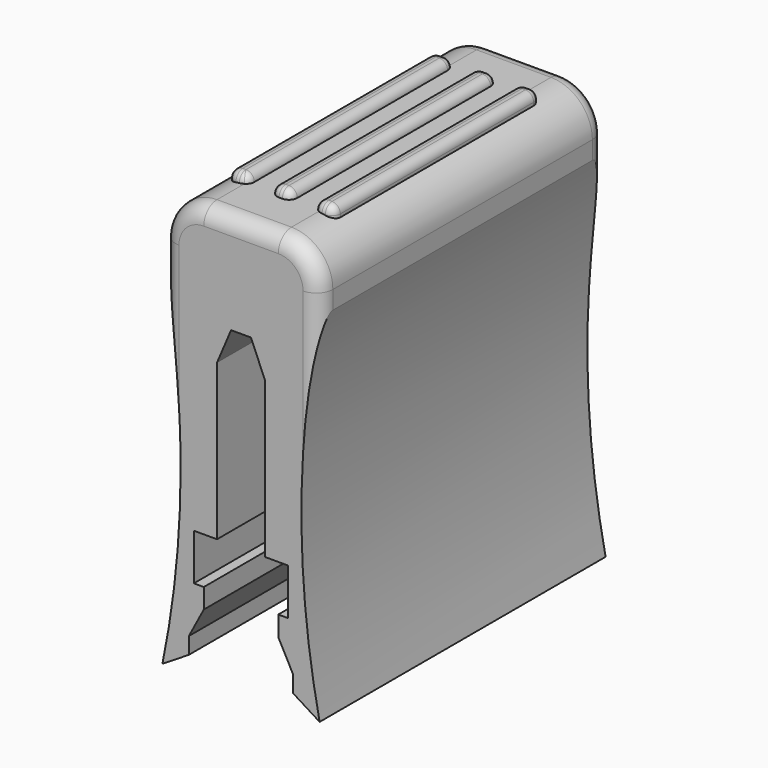
from build123d import *

# Parameters (mm, degrees)
F1_DEPTH = 21.6
F2_R     = 1
F4_DEPTH = 0.5
F5_R     = 0.49999


# Not quite as in the source:
# - a fillet or chamfer is up to 0.001 mm smaller than in the source, because OpenCascade refuses the exact size


with BuildPart() as f1:
    # F0 (on Front) → F1 (new body)
    with BuildSketch(Plane.XZ):
        with BuildLine():
            ThreePointArc((4.75, 10.05), (4.017766953, 11.817766953), (2.25, 12.55))
            Line((2.25, 12.55), (-2.25, 12.55))
            ThreePointArc((-2.25, 12.55), (-4.017766953, 11.817766953), (-4.75, 10.05))
            Line((-4.75, 10.05), (-4.75, 8.95))
            ThreePointArc((-4.75, 8.95), (-3.9257161045, 3.6030662591), (-3.65, -1.8))
            ThreePointArc((-3.65, -1.8), (-3.9257161045, -7.2030662591), (-4.75, -12.55))
            Line((-4.75, -12.55), (-3.15, -11.55))
            Line((-3.15, -11.55), (-3.15, -10.55))
            Line((-3.15, -10.55), (-2.25, -8.85))
            Line((-2.25, -8.85), (-2.25, -7.65))
            Line((-2.25, -7.65), (-2.85, -7.65))
            Line((-2.85, -7.65), (-2.85, -4.85))
            Line((-2.85, -4.85), (-1.45, -4.85))
            Line((-1.45, -4.85), (-1.45, 4.55))
            Line((-1.45, 4.55), (-0.6, 6.55))
            Line((-0.6, 6.55), (0, 6.55))
            Line((0, 6.55), (0.6, 6.55))
            Line((0.6, 6.55), (1.45, 4.55))
            Line((1.45, 4.55), (1.45, -4.85))
            Line((1.45, -4.85), (2.85, -4.85))
            Line((2.85, -4.85), (2.85, -7.65))
            Line((2.85, -7.65), (2.25, -7.65))
            Line((2.25, -7.65), (2.25, -8.85))
            Line((2.25, -8.85), (3.15, -10.55))
            Line((3.15, -10.55), (3.15, -11.55))
            Line((3.15, -11.55), (4.75, -12.55))
            ThreePointArc((4.75, -12.55), (3.65, -1.8), (4.75, 8.95))
            Line((4.75, 8.95), (4.75, 10.05))
        make_face()
    extrude(amount=F1_DEPTH)

    # F2
    f2_edges = [f1.edges().sort_by_distance(p)[0] for p in [
        (0, 0, 12.55),
        (0, -21.6, 12.55),
    ]]
    fillet(f2_edges, radius=F2_R)

    # F3 (on face) → F4 (join, symmetric)
    with BuildSketch(Plane.XY.offset(12.55)):
        with BuildLine():
            ThreePointArc((2.5, -3), (2.3705904774, -3.0170370869), (2.25, -3.0669872981))
            Line((2.25, -3.0669872981), (2.25, -18.5330127019))
            ThreePointArc((2.25, -18.5330127019), (2.3705904774, -18.5829629131), (2.5, -18.6))
            Line((2.5, -18.6), (2.7, -18.6))
            ThreePointArc((2.7, -18.6), (3.0535533906, -18.4535533906), (3.2, -18.1))
            Line((3.2, -18.1), (3.2, -3.5))
            ThreePointArc((3.2, -3.5), (3.0535533906, -3.1464466094), (2.7, -3))
            Line((2.7, -3), (2.5, -3))
        make_face()
        with BuildLine():
            Line((2.25, -18.5330127019), (2.25, -3.0669872981))
            ThreePointArc((2.25, -3.0669872981), (2.0669872981, -3.25), (2, -3.5))
            Line((2, -3.5), (2, -18.1))
            ThreePointArc((2, -18.1), (2.0669872981, -18.35), (2.25, -18.5330127019))
        make_face()
        with BuildLine():
            Line((0.1, -3), (-0.1, -3))
            ThreePointArc((-0.1, -3), (-0.4535533906, -3.1464466094), (-0.6, -3.5))
            Line((-0.6, -3.5), (-0.6, -18.1))
            ThreePointArc((-0.6, -18.1), (-0.4535533906, -18.4535533906), (-0.1, -18.6))
            Line((-0.1, -18.6), (0.1, -18.6))
            ThreePointArc((0.1, -18.6), (0.4535533906, -18.4535533906), (0.6, -18.1))
            Line((0.6, -18.1), (0.6, -3.5))
            ThreePointArc((0.6, -3.5), (0.4535533906, -3.1464466094), (0.1, -3))
        make_face()
        with BuildLine():
            Line((-2, -18.1), (-2, -3.5))
            ThreePointArc((-2, -3.5), (-2.0669872981, -3.25), (-2.25, -3.0669872981))
            Line((-2.25, -3.0669872981), (-2.25, -18.5330127019))
            ThreePointArc((-2.25, -18.5330127019), (-2.0669872981, -18.35), (-2, -18.1))
        make_face()
        with BuildLine():
            Line((-2.25, -18.5330127019), (-2.25, -3.0669872981))
            ThreePointArc((-2.25, -3.0669872981), (-2.3705904774, -3.0170370869), (-2.5, -3))
            Line((-2.5, -3), (-2.7, -3))
            ThreePointArc((-2.7, -3), (-3.0535533906, -3.1464466094), (-3.2, -3.5))
            Line((-3.2, -3.5), (-3.2, -18.1))
            ThreePointArc((-3.2, -18.1), (-3.0535533906, -18.4535533906), (-2.7, -18.6))
            Line((-2.7, -18.6), (-2.5, -18.6))
            ThreePointArc((-2.5, -18.6), (-2.3705904774, -18.5829629131), (-2.25, -18.5330127019))
        make_face()
    extrude(amount=F4_DEPTH, both=True)

    # F5 (radius 0.5 in the source; OpenCascade refuses exactly that, so slightly less here)
    f5_edges = [f1.edges().sort_by_distance(p)[0] for p in [
        (-2, -10.8, 13.05),
        (-2.146447, -3.146447, 13.05),
        (-2.6, -3, 13.05),
        (-3.053553, -3.146447, 13.05),
        (-3.2, -10.8, 13.05),
        (-3.053553, -18.453553, 13.05),
        (-2.6, -18.6, 13.05),
        (-2.146447, -18.453553, 13.05),
        (0.6, -10.8, 13.05),
        (0.453553, -3.146447, 13.05),
        (0, -3, 13.05),
        (-0.453553, -3.146447, 13.05),
        (-0.6, -10.8, 13.05),
        (-0.453553, -18.453553, 13.05),
        (0, -18.6, 13.05),
        (0.453553, -18.453553, 13.05),
        (2.146447, -3.146447, 13.05),
        (2, -10.8, 13.05),
        (2.146447, -18.453553, 13.05),
        (2.6, -18.6, 13.05),
        (3.053553, -18.453553, 13.05),
        (3.2, -10.8, 13.05),
        (3.053553, -3.146447, 13.05),
        (2.6, -3, 13.05),
    ]]
    fillet(f5_edges, radius=F5_R)


solid = f1.part
